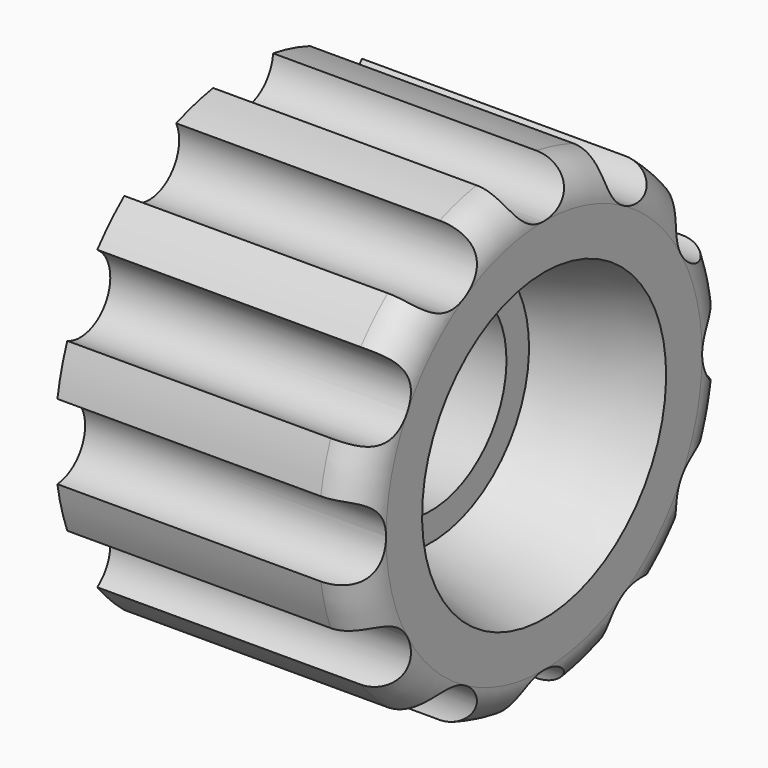
from build123d import *

# Parameters (mm, degrees)
F2_R     = 4.0538475773
F3_DEPTH = 8
F4_R     = 0.99999


# Not quite as in the source:
# - a fillet or chamfer is up to 0.001 mm smaller than in the source, because OpenCascade refuses the exact size


with BuildPart() as f1:
    # F0 (on Front) → F1 (revolve)
    with BuildSketch(Plane.XZ):
        Polygon((0, 4.0538475773), (0, 2.5), (5, 2.5), (5, 3.25), (8, 4.0538475773), align=None)
    revolve(axis=Axis((3.9731631987, 0, 0), (1, 0, 0)))

    # F2 (on Right) → F3 (join)
    with BuildSketch(Plane.YZ):
        with BuildLine():
            ThreePointArc((-2.2217503258, 5.8417741731), (-2.625, 4.5466333699), (-3.9482496742, 4.8449793096))
            ThreePointArc((-3.9482496742, 4.8449793096), (-4.4194173824, 4.4194173824), (-4.8449793096, 3.9482496742))
            ThreePointArc((-4.8449793096, 3.9482496742), (-4.5466333699, 2.625), (-5.8417741731, 2.2217503258))
            ThreePointArc((-5.8417741731, 2.2217503258), (-6.0370364143, 1.6176190319), (-6.17, 0.9967948636))
            ThreePointArc((-6.17, 0.9967948636), (-5.25, 0), (-6.17, -0.9967948636))
            ThreePointArc((-6.17, -0.9967948636), (-6.0370364143, -1.6176190319), (-5.8417741731, -2.2217503258))
            ThreePointArc((-5.8417741731, -2.2217503258), (-4.5466333699, -2.625), (-4.8449793096, -3.9482496742))
            ThreePointArc((-4.8449793096, -3.9482496742), (-4.4194173824, -4.4194173824), (-3.9482496742, -4.8449793096))
            ThreePointArc((-3.9482496742, -4.8449793096), (-2.625, -4.5466333699), (-2.2217503258, -5.8417741731))
            ThreePointArc((-2.2217503258, -5.8417741731), (-1.6176190319, -6.0370364143), (-0.9967948636, -6.17))
            ThreePointArc((-0.9967948636, -6.17), (0, -5.25), (0.9967948636, -6.17))
            ThreePointArc((0.9967948636, -6.17), (1.6176190319, -6.0370364143), (2.2217503258, -5.8417741731))
            ThreePointArc((2.2217503258, -5.8417741731), (2.625, -4.5466333699), (3.9482496742, -4.8449793096))
            ThreePointArc((3.9482496742, -4.8449793096), (4.4194173824, -4.4194173824), (4.8449793096, -3.9482496742))
            ThreePointArc((4.8449793096, -3.9482496742), (4.5466333699, -2.625), (5.8417741731, -2.2217503258))
            ThreePointArc((5.8417741731, -2.2217503258), (6.0370364143, -1.6176190319), (6.17, -0.9967948636))
            ThreePointArc((6.17, -0.9967948636), (5.25, 0), (6.17, 0.9967948636))
            ThreePointArc((6.17, 0.9967948636), (6.0370364143, 1.6176190319), (5.8417741731, 2.2217503258))
            ThreePointArc((5.8417741731, 2.2217503258), (4.5466333699, 2.625), (4.8449793096, 3.9482496742))
            ThreePointArc((4.8449793096, 3.9482496742), (4.4194173824, 4.4194173824), (3.9482496742, 4.8449793096))
            ThreePointArc((3.9482496742, 4.8449793096), (2.625, 4.5466333699), (2.2217503258, 5.8417741731))
            ThreePointArc((2.2217503258, 5.8417741731), (1.6176190319, 6.0370364143), (0.9967948636, 6.17))
            ThreePointArc((0.9967948636, 6.17), (0, 5.25), (-0.9967948636, 6.17))
            ThreePointArc((-0.9967948636, 6.17), (-1.6176190319, 6.0370364143), (-2.2217503258, 5.8417741731))
        make_face()
        Circle(F2_R, mode=Mode.SUBTRACT)
    extrude(amount=F3_DEPTH)

    # F4 (radius 1 in the source; OpenCascade refuses exactly that, so slightly less here)
    f4_edges = [f1.edges().sort_by_distance(p)[0] for p in [
        (8, -4.419417, 4.419417),
        (8, -1.617619, 6.037036),
        (8, 1.617619, 6.037036),
        (8, 4.419417, 4.419417),
        (8, 6.037036, 1.617619),
        (8, 6.037036, -1.617619),
        (8, 4.419417, -4.419417),
        (8, 1.617619, -6.037036),
        (8, -1.617619, -6.037036),
        (8, -4.419417, -4.419417),
        (8, -6.037036, -1.617619),
        (8, -6.037036, 1.617619),
    ]]
    fillet(f4_edges, radius=F4_R)


solid = f1.part
